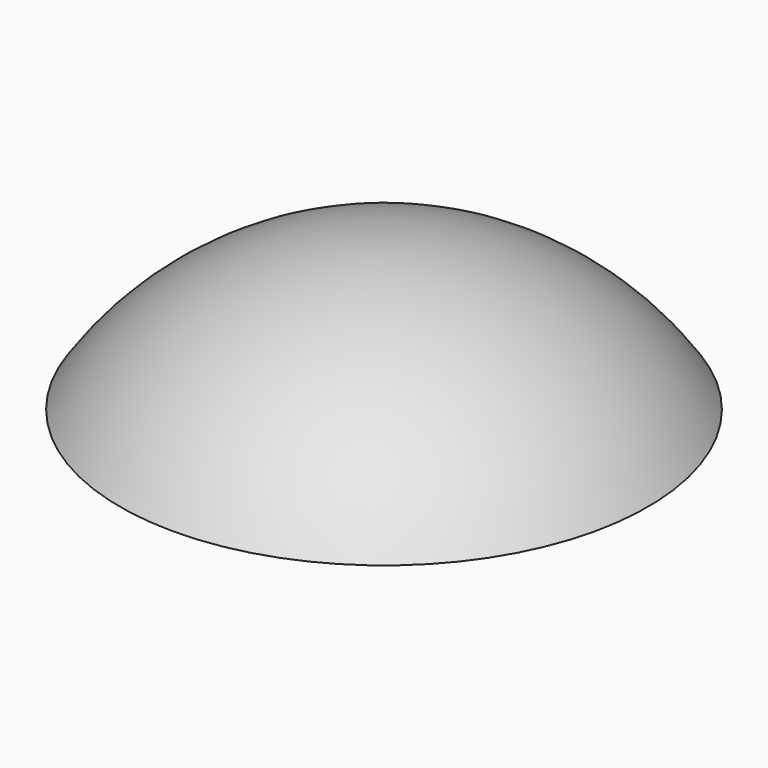
from build123d import *

# Parameters (mm, degrees)
F3_T     = -2.54
F4_R     = 3.81
F4_R_2   = 1.3335
F6_R     = 1.27
F7_R     = 18.415
F8_DEPTH = 10.16


with BuildPart() as f2:
    # F1 (on Right) → F2 (revolve)
    with BuildSketch(Plane.YZ):
        with BuildLine():
            Line((0, 18.415), (0, 0))
            Line((0, 0), (18.415, 0))
            ThreePointArc((18.415, 0), (13.0213713756, 13.0213713756), (0, 18.415))
        make_face()
    revolve(axis=Axis((0, 0, 9.2075), (0, 0, 1)))

    # F3
    f3_openings = [f2.faces().sort_by_distance(p)[0] for p in [
        (0, 0, 0),
    ]]
    offset(amount=F3_T, openings=f3_openings)

    # F4 (on face) → F5 (join, up to the next surface of F2)
    with BuildSketch(Plane.XY):
        Circle(F4_R)
        Circle(F4_R_2, mode=Mode.SUBTRACT)
    extrude(until=Until.NEXT)

    # F6
    f6_edges = [f2.edges().sort_by_distance(p)[0] for p in [
        (-2.694077, -2.694077, 15.41102),
        (2.694077, 2.694077, 15.41102),
    ]]
    fillet(f6_edges, radius=F6_R)

    # F7 (on face) → F8 (cut)
    with BuildSketch(Plane.XY):
        Circle(F7_R)
    extrude(amount=F8_DEPTH, mode=Mode.SUBTRACT)


solid = f2.part
